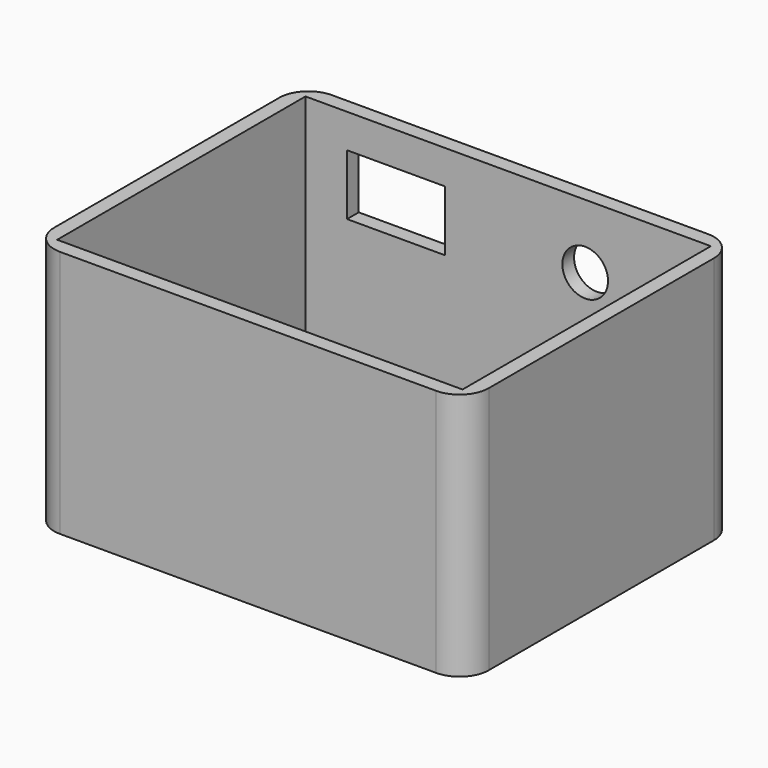
from build123d import *

# Parameters (mm, degrees)
F0_W     = 75.565
F0_H     = 59.055
F1_DEPTH = 43.18
F2_T     = -2.54
F3_W     = 17.018
F3_H     = 10.541
F4_DEPTH = 3.302
F6_D     = 7.9375
F6_DEPTH = 12.7
F6_TIP   = 2.3846655818
F7_R     = 5.08


# Not quite as in the source:
# - a feature names something its author has since deleted; it is built from what else it names


with BuildPart() as f1:
    # F0 (on Top) → F1 (new body)
    with BuildSketch(Plane.XY):
        Rectangle(F0_W, F0_H)
    extrude(amount=F1_DEPTH)

    # F2
    f2_openings = [f1.faces().sort_by_distance(p)[0] for p in [
        (0, 0, 43.18),
    ]]
    offset(amount=F2_T, openings=f2_openings)

    # F3 (on face) → F4 (cut)
    with BuildSketch(Plane(origin=(0, 29.5275, 0), x_dir=(-1, 0, 0), z_dir=(0, 1, 0))):
        with Locations((19.5056423545, 32.0256687701)):
            Rectangle(F3_W, F3_H)
    extrude(amount=-F4_DEPTH, mode=Mode.SUBTRACT)

    # F6
    with Locations(Plane(origin=(0, 29.5275, 0), x_dir=(-1, 0, 0), z_dir=(0, 1, 0))):
        with Locations((-13.3929288228, 32.0256687701)):
            Hole(F6_D / 2, depth=F6_DEPTH)
            with Locations((0, 0, -(F6_DEPTH + F6_TIP / 2))):  # 118° drill point
                Cone(0, F6_D / 2, F6_TIP, mode=Mode.SUBTRACT)

    # F7
    f7_edges = [f1.edges().sort_by_distance(p)[0] for p in [
        (-37.7825, -29.5275, 21.59),
        (37.7825, -29.5275, 21.59),
        (37.7825, 29.5275, 21.59),
        (-37.7825, 29.5275, 21.59),
    ]]
    fillet(f7_edges, radius=F7_R)


solid = f1.part
